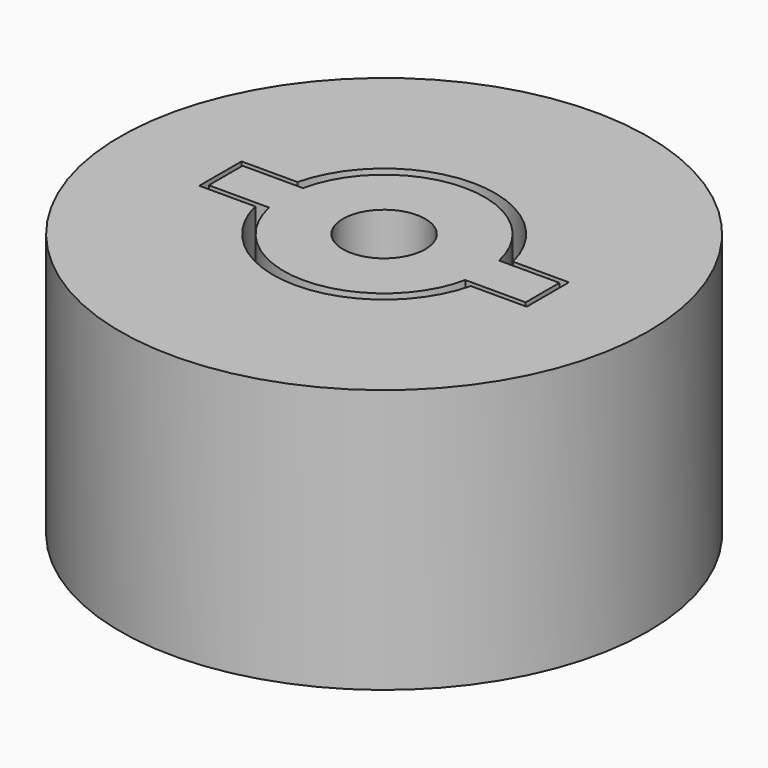
from build123d import *

# Parameters (mm, degrees)
F0_R      = 25
F0_R_2    = 10.5055534995
F1_DEPTH  = 25
F2_DEPTH  = 7
F3_D      = 6.8
F3_DEPTH  = 12.25
F3_TIP    = 2.0429261047
F5_DEPTH  = 10
F7_DEPTH  = 9
F9_DEPTH  = 16
F10_R     = 3.9
F11_DEPTH = 10
F12_DEPTH = 25


with BuildPart() as f1:
    # F0 (on Top) → F1 (new body)
    with BuildSketch(Plane.XY):
        Circle(F0_R)
        Circle(F0_R_2, mode=Mode.SUBTRACT)
    extrude(amount=F1_DEPTH)

    # F4 (on face) → F5 (cut)
    with BuildSketch(Plane.XY.offset(25)):
        with BuildLine():
            Line((-10.2037568733, 2.5), (-15.5055534995, 2.5))
            Line((-15.5055534995, 2.5), (-15.5055534995, -2.5))
            Line((-15.5055534995, -2.5), (-10.2037568733, -2.5))
            ThreePointArc((-10.2037568733, -2.5), (-10.5055534995, 0), (-10.2037568733, 2.5))
        make_face()
        with BuildLine():
            Line((15.5055534995, 2.5), (10.2037568733, 2.5))
            ThreePointArc((10.2037568733, 2.5), (10.4298314478, 1.2590751768), (10.5055534995, 0))
            ThreePointArc((10.5055534995, 0), (10.4298314478, -1.2590751768), (10.2037568733, -2.5))
            Line((10.2037568733, -2.5), (15.5055534995, -2.5))
            Line((15.5055534995, -2.5), (15.5055534995, 2.5))
        make_face()
    extrude(amount=-F5_DEPTH, mode=Mode.SUBTRACT)


with BuildPart() as f2:
    # F0 (on Top) → F2 (new body)
    with BuildSketch(Plane.XY):
        Polygon((3.7527767497, 6.5), (-3.7527767497, 6.5), (-7.5055534995, 0), (-3.7527767497, -6.5), (3.7527767497, -6.5), (7.5055534995, 0), align=None)
    extrude(amount=F2_DEPTH)

    # F3
    with Locations(Plane(origin=(0, 0, 0), x_dir=(1, 0, 0), z_dir=(0, 0, -1))):
        with Locations((0, 0)):
            Hole(F3_D / 2, depth=F3_DEPTH)
            with Locations((0, 0, -(F3_DEPTH + F3_TIP / 2))):  # 118° drill point
                Cone(0, F3_D / 2, F3_TIP, mode=Mode.SUBTRACT)


with BuildPart() as f7:
    # F6 (on face) → F7 (new body, through all)
    with BuildSketch(Plane.XY.offset(25)):
        with BuildLine():
            Line((-15.0055534995, -2), (-9.2927685504, -2))
            ThreePointArc((-9.2927685504, -2), (0, -9.5055534995), (9.2927685504, -2))
            Line((9.2927685504, -2), (15.0055534995, -2))
            Line((15.0055534995, -2), (15.0055534995, 2))
            Line((15.0055534995, 2), (9.2927685504, 2))
            ThreePointArc((9.2927685504, 2), (0, 9.5055534995), (-9.2927685504, 2))
            Line((-9.2927685504, 2), (-15.0055534995, 2))
            Line((-15.0055534995, 2), (-15.0055534995, -2))
        make_face()
    extrude(amount=-F7_DEPTH)

    # F8 (on face) → F9 (join, through all)
    with BuildSketch(Plane(origin=(0, 0, 16), x_dir=(1, 0, 0), z_dir=(0, 0, -1))):
        with BuildLine():
            ThreePointArc((9.2927685504, -2), (9.4522075714, -1.0056437533), (9.5055534995, 0))
            ThreePointArc((9.5055534995, 0), (9.4522075714, 1.0056437533), (9.2927685504, 2))
            ThreePointArc((9.2927685504, 2), (0, 9.5055534995), (-9.2927685504, 2))
            ThreePointArc((-9.2927685504, 2), (-9.5055534995, 0), (-9.2927685504, -2))
            ThreePointArc((-9.2927685504, -2), (0, -9.5055534995), (9.2927685504, -2))
        make_face()
    extrude(amount=F9_DEPTH)

    # F10 (on face) → F11 (cut)
    with BuildSketch(Plane(origin=(0, 0, 0), x_dir=(1, 0, 0), z_dir=(0, 0, -1))):
        Polygon((8.0829037687, 0), (4.0414518843, 7), (-4.0414518843, 7), (-8.0829037687, 0), (-4.0414518843, -7), (4.0414518843, -7), align=None)
        Polygon((-7.5055534995, 0), (-3.7527767497, 6.5), (3.7527767497, 6.5), (7.5055534995, 0), (3.7527767497, -6.5), (-3.7527767497, -6.5), align=None, mode=Mode.SUBTRACT)
        Polygon((3.7527767497, 6.5), (-3.7527767497, 6.5), (-7.5055534995, 0), (-3.7527767497, -6.5), (3.7527767497, -6.5), (7.5055534995, 0), align=None)
        Circle(F10_R, mode=Mode.SUBTRACT)
        Circle(F10_R)
    extrude(amount=-F11_DEPTH, mode=Mode.SUBTRACT)

    # F10 (on face) → F12 (cut, through all)
    with BuildSketch(Plane(origin=(0, 0, 0), x_dir=(1, 0, 0), z_dir=(0, 0, -1))):
        Circle(F10_R)
    extrude(amount=-F12_DEPTH, mode=Mode.SUBTRACT)


solid = Compound([f1.part, f2.part, f7.part])
